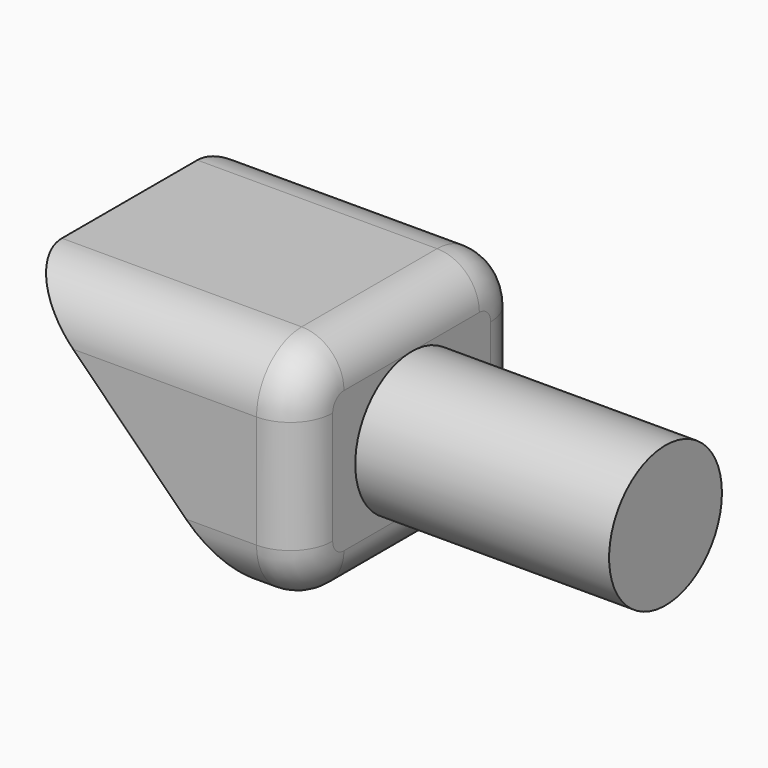
from build123d import *

# Parameters (mm, degrees)
F0_W     = 10
F0_H     = 8
F1_DEPTH = 5
F3_DEPTH = 10.001
F4_R     = 2.5
F5_DEPTH = 9
F6_R     = 2
F7_R     = 1.49999


# Not quite as in the source:
# - a fillet or chamfer is up to 0.001 mm smaller than in the source, because OpenCascade refuses the exact size


with BuildPart() as f1:
    # F0 (on Front) → F1 (new body, symmetric)
    with BuildSketch(Plane.XZ):
        Rectangle(F0_W, F0_H)
    extrude(amount=F1_DEPTH, both=True)

    # F2 (on face) → F3 (cut, through all)
    with BuildSketch(Plane.XZ.offset(5)):
        Polygon((3, -4), (-5, 4), (-5, -4), align=None)
    extrude(amount=-F3_DEPTH, mode=Mode.SUBTRACT)

    # F4 (on face) → F5 (join)
    with BuildSketch(Plane.YZ.offset(5)):
        Circle(F4_R)
    extrude(amount=F5_DEPTH)

    # F6
    f6_edges = [f1.edges().sort_by_distance(p)[0] for p in [
        (0, -5, 4),
        (0, 5, 4),
        (4, -5, -4),
        (4, 5, -4),
    ]]
    fillet(f6_edges, radius=F6_R)

    # F7 (radius 1.5 in the source; OpenCascade refuses exactly that, so slightly less here)
    f7_edges = [f1.edges().sort_by_distance(p)[0] for p in [
        (5, -5, 0),
    ]]
    fillet(f7_edges, radius=F7_R)


solid = f1.part
